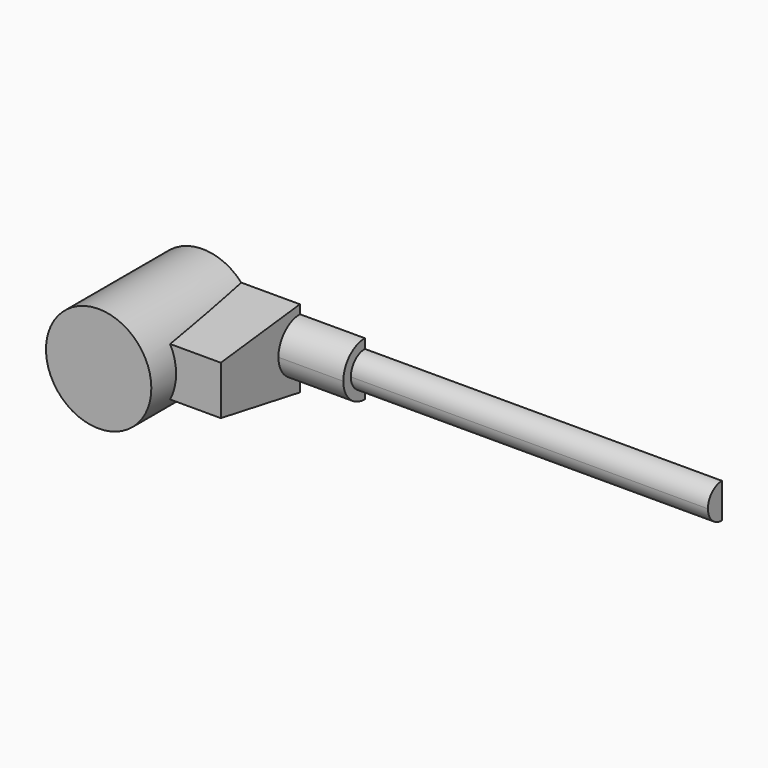
from build123d import *

# Parameters (mm, degrees)
F0_R     = 8.1133177019
F1_DEPTH = 20
F3_DEPTH = 15
F5_DEPTH = 25
F7_DEPTH = 80


# Not quite as in the source:
# - a feature names something its author has since deleted; it is built from what else it names


with BuildPart() as f1:
    # F0 (on Front) → F1 (new body)
    with BuildSketch(Plane.XZ):
        Circle(F0_R)
    extrude(amount=F1_DEPTH)

    # F2 (on Right) → F3 (join)
    with BuildSketch(Plane.YZ):
        Polygon((0, -6.4580785111), (0, 5.4941866547), (-15.2294980362, 3.7591799628), (-15.2294980362, -3.7591799628), align=None)
    extrude(amount=F3_DEPTH)

    # F4 (on Right) → F5 (join)
    with BuildSketch(Plane.YZ):
        with BuildLine():
            ThreePointArc((-4.1447370313, 0), (-2.9307716611, -2.9307716611), (0, -4.1447370313))
            Line((0, -4.1447370313), (0, 4.1447370313))
            ThreePointArc((0, 4.1447370313), (-2.9307716611, 2.9307716611), (-4.1447370313, 0))
        make_face()
    extrude(amount=F5_DEPTH)

    # F6 (on Right) → F7 (join)
    with BuildSketch(Plane.YZ):
        with BuildLine():
            ThreePointArc((-2.6943630073, 0), (-1.9052023535, -1.9052023535), (0, -2.6943630073))
            Line((0, -2.6943630073), (0, 2.6943630073))
            ThreePointArc((0, 2.6943630073), (-1.9052023535, 1.9052023535), (-2.6943630073, 0))
        make_face()
    extrude(amount=F7_DEPTH)


solid = f1.part
